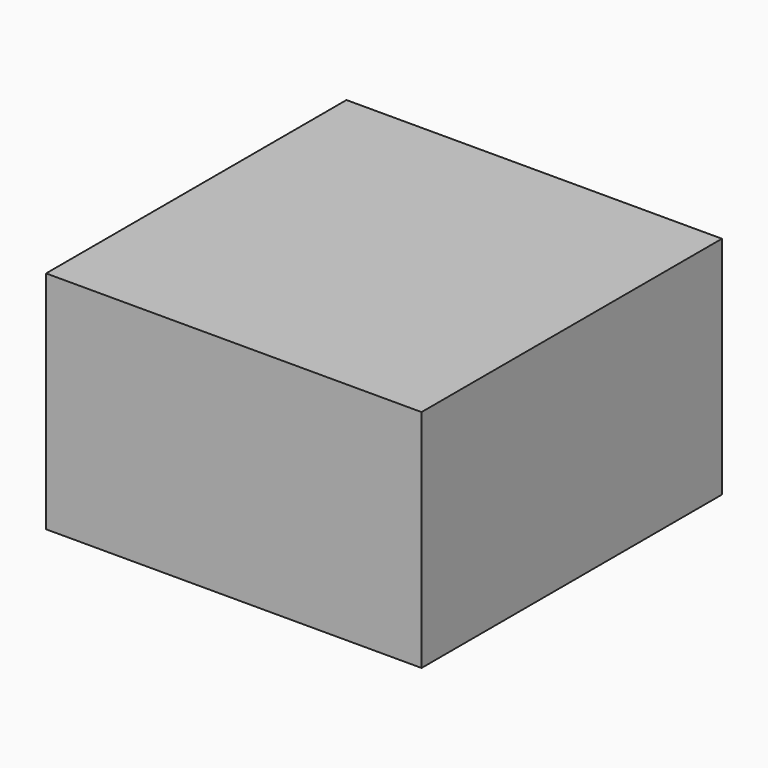
from build123d import *

# Parameters (mm, degrees)
F4_W     = 50
F4_H     = 50
F5_DEPTH = 30


with BuildPart() as f5:
    # F4 (on Top) → F5 (new body)
    with BuildSketch(Plane.XY):
        with Locations((25, 25)):
            Rectangle(F4_W, F4_H)
    extrude(amount=-F5_DEPTH)

    # F1 (on Front) → F6 section 0
    with BuildSketch(Plane.XZ):
        with BuildLine():
            Line((40, 0), (10, 0))
            Line((10, 0), (28.3937944681, -18.3937944681))
            ThreePointArc((28.3937944681, -18.3937944681), (33.3782491174, -19.6437206946), (36.8322317524, -15.8388412378))
            Line((36.8322317524, -15.8388412378), (40, 0))
        make_face()
    # F3 (on offset) → F6 section 1
    with BuildSketch(Plane.YZ.offset(50)):
        with BuildLine():
            Line((40, 0), (10, 0))
            Line((10, 0), (24.3103555535, -8.5862133321))
            ThreePointArc((24.3103555535, -8.5862133321), (32.9247755851, -9.390134224), (38.9421460883, -3.1735617351))
            Line((38.9421460883, -3.1735617351), (40, 0))
        make_face()
    loft()


solid = f5.part
